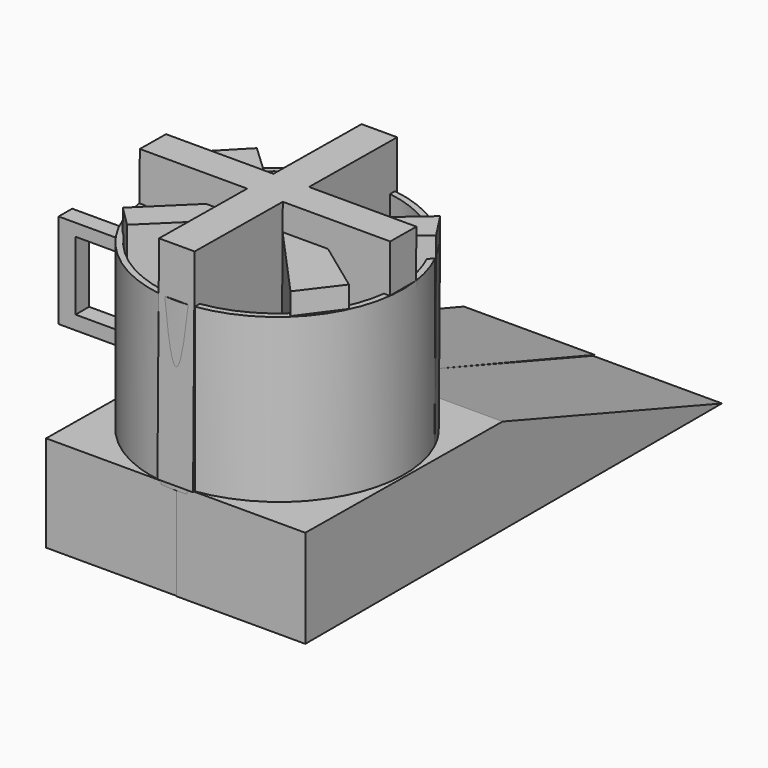
from build123d import *
from build123d import SkipClean  # not in build123d's __all__

# Parameters (mm, degrees)
F0_W         = 53.0167296529
F0_H         = 70.1501816511
F2_W         = 33.9436382055
F2_H         = 39.762545377
F2_W_2       = 20.6894539297
F2_H_2       = 28.7712737918
F3_DEPTH     = 7.112
F4_T         = 2.54
F4_T3_DEPTH  = 44.842545377
F4_T5_DEPTH  = 12.192
F4_T8_ANGLE  = 7.7092595128
F4_T10_ANGLE = 7.7092595128
F6_DEPTH     = 54.102
F8_DEPTH     = 54.864
F9_W         = 14.9403763935
F9_H         = 46.2447360097
F9_W_2       = 45.0574515454
F9_H_2       = 13.7577369931
F10_DEPTH    = 88.646
F12_DEPTH    = 77.47


# Not quite as in the source:
# - a shell that OpenCascade refuses in one call is made with other operations: the cavity is built on its own and cut out


with BuildPart() as f1:
    # F0 (on Front) → F1 (revolve)
    with BuildSketch(Plane.XZ):
        with Locations((-26.5083648264, 0.9679794312)):
            Rectangle(F0_W, F0_H)
    revolve(axis=Axis((0, 0, 0.9679794312), (0, 0, 1)))

    # F2 (on Front) → F3 (join)
    with BuildSketch(Plane.XZ):
        with Locations((-69.0187290311, 0.6447080523)):
            Rectangle(F2_W, F2_H)
        with Locations((-68.5338173062, 0.9679803625)):
            Rectangle(F2_W_2, F2_H_2, mode=Mode.SUBTRACT)
    extrude(amount=F3_DEPTH)

    # F4: shell of thickness 2.54, made by hand


with BuildPart() as f4_core1:
    # F4_t2: copy of F1
    add(f1.part, clean=False)

    # the walls: a layer under each face that stays
    f4_faces = [f4_core1.faces().sort_by_distance(p)[0] for p in [
        (0, 0, -34.1071113944),
        (53.0167296529, 0, 0.9679794312),
        (-69.2640439234, -3.556, 20.5259807408),
        (-80.4150467304, -7.112, -12.6094737401),
        (-69.2640439234, -3.556, -19.2365646362),
        (-80.4949117204, 0, -12.6094737401),
        (-85.9905481339, -3.556, 0.6447080523),
        (-68.5338173062, -3.556, 15.3536172584),
        (-78.878544271, -3.556, 0.9679803625),
        (-58.1890903413, -3.556, 0.9679803625),
        (-68.5338173062, -3.556, -13.4176565334),
    ]]
    thicken(f4_faces, amount=-F4_T, mode=Mode.SUBTRACT)

    # F4_s4 → F4_t3 (cut)
    with BuildSketch(Plane.XY.offset(-21.7765646362)):
        Polygon((-52.5627101359, -7.1408073169), (-50.0204974181, -6.771268308), (-50.3182120863, -4.572), (-52.5375397129, -4.572), align=None)
        Polygon((-53.0421296529, 0.0254), (-50.4767296529, 0), (-50.4767296529, -2.54), (-53.0167296529, -2.54), align=None)
    extrude(amount=F4_T3_DEPTH, mode=Mode.SUBTRACT)

    # F4_s6 → F4_t5 (cut)
    with BuildSketch(Plane.XZ.offset(-2.54)):
        Polygon((-78.853144271, 15.3282172584), (-78.878544271, 17.8936172584), (-81.418544271, 17.8936172584), (-81.418544271, 15.3536172584), align=None)
        Polygon((-58.2144903413, 15.3282172584), (-58.1890903413, 17.8936172584), (-55.6490903413, 17.8936172584), (-55.6490903413, 15.3536172584), align=None)
        Polygon((-78.853144271, -13.3922565334), (-81.418544271, -13.4176565334), (-81.418544271, -15.9576565334), (-78.878544271, -15.9576565334), align=None)
        Polygon((-58.2144903413, -13.3922565334), (-55.6490903413, -13.4176565334), (-55.6490903413, -15.9576565334), (-58.1890903413, -15.9576565334), align=None)
    extrude(amount=F4_T5_DEPTH, mode=Mode.SUBTRACT)

    # F4_s7 → F4_t8 (revolve, cut)
    with BuildSketch(Plane(origin=(0, 0, 0), x_dir=(0, 0, 1), z_dir=(0.1341463354, -0.9909615334, 0))):
        Polygon((20.5513807408, 53.0421296529), (20.5259807408, 50.4767296529), (17.9859807408, 50.4767296529), (17.9859807408, 53.0167296529), align=None)
    revolve(axis=Axis((0, 0, 20.5259807408), (0, 0, -1)), revolution_arc=F4_T8_ANGLE, mode=Mode.SUBTRACT)

    # F4_s9 → F4_t10 (revolve, cut)
    with BuildSketch(Plane(origin=(0, 0, 0), x_dir=(0, 0, 1), z_dir=(0.1341463354, -0.9909615334, 0))):
        Polygon((-19.2619646362, 53.0421296529), (-19.2365646362, 50.4767296529), (-16.6965646362, 50.4767296529), (-16.6965646362, 53.0167296529), align=None)
    revolve(axis=Axis((0, 0, -19.2365646362), (0, 0, -1)), revolution_arc=F4_T10_ANGLE, mode=Mode.SUBTRACT)


with BuildPart() as f1_1:
    add(f1.part, clean=False)

    # what is left inside the walls is the cavity
    f4_cavity = [f4_core1.part.solids().sort_by_distance(p)[0] for p in [
        (50.3372, 3.391603, 13.506343),
    ]]
    add(f4_cavity, mode=Mode.SUBTRACT)

    # F5 (on Right) → F6 (join)
    with BuildSketch(Plane.YZ):
        Polygon((50.610627979, -33.1372953951), (-52.8366453946, -32.1674756706), (-52.8366453946, -73.2231140137), (165.6957119703, -73.2231140137), align=None)
    extrude(amount=F6_DEPTH)

    # F7 (on Right) → F8 (join)
    with BuildSketch(Plane.YZ):
        Polygon((52.1392673254, -33.7838381529), (-52.6010990143, -32.8140184283), (-52.6010990143, -73.2231140137), (166.5778160095, -73.2231140137), align=None)
    extrude(amount=-F8_DEPTH)

    # F9 (on face) → F10 (join)
    with BuildSketch(Plane(origin=(0, -0.3061875117, -32.6599494936), x_dir=(1, 0, 0), z_dir=(0, 0.0093746029, 0.9999560574))):
        with Locations((0, -30.0012365014)):
            Rectangle(F9_W, F9_H)
        with Locations((-29.9989139694, 0)):
            Rectangle(F9_W_2, F9_H_2)
        Rectangle(F9_W, F9_H_2)
        with Locations((29.9989139694, 0)):
            Rectangle(F9_W_2, F9_H_2)
        with Locations((0, 30.0012365014)):
            Rectangle(F9_W, F9_H)
    with SkipClean():  # cleaning this boolean's faces spoils the solid; the shape is the same uncleaned
        extrude(amount=F10_DEPTH)

    # F11 (on face) → F12 (join)
    with BuildSketch(Plane(origin=(0, -0.3061875117, -32.6599494936), x_dir=(1, 0, 0), z_dir=(0, 0.0093746029, 0.9999560574))):
        Polygon((-35.2792814374, -35.0489541888), (-6.9552087225, -6.723633036), (7.4701881967, -6.8788684965), (-9.015141055, 8.7265400216), (-36.82423383, 34.9918417633), (-47.9992774731, 23.1599645401), (-27.8100166411, 4.0914881974), (-22.4047969755, -4.6636964383), (-44.0343843394, -26.2942371678), align=None)
        Polygon((9.0424474554, 7.2099834745), (7.4701881967, -6.8788684965), (36.0927975577, -38.5295574829), (47.8385306477, -22.5475626063), (26.5187043697, -6.8788684965), (26.5187043697, 4.0914881974), (47.8385306477, 23.1599645401), (40.2370781386, 34.8294671803), align=None)
        Polygon((-9.015141055, 8.7265400216), (7.4701881967, -6.8788684965), (9.0424474554, 7.2099834745), align=None)
    with SkipClean():  # cleaning this boolean's faces spoils the solid; the shape is the same uncleaned
        extrude(amount=F12_DEPTH)


solid = f1_1.part
